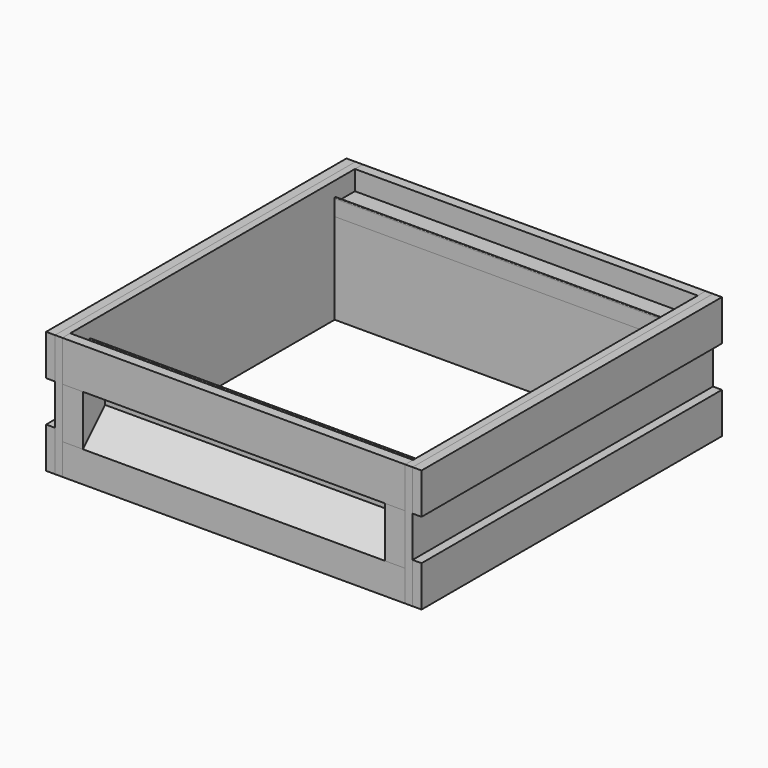
from build123d import *

# Parameters (mm, degrees)
F0_W      = 9
F0_H      = 126
F1_DEPTH  = 210
F2_W      = 34
F2_H      = 38
F3_DEPTH  = 210
F5_DEPTH  = 420
F9_DEPTH  = 9
F10_W     = 11
F10_H     = 50
F11_DEPTH = 460
F12_W     = 34
F12_H     = 62
F13_DEPTH = 25
F16_DEPTH = 370


# Not quite as in the source:
# - ends of sketch curves that miss each other by under 0.0002 mm in the source are joined


with BuildPart() as f1:
    # F0 (on Right) → F1 (new body, symmetric)
    with BuildSketch(Plane.YZ):
        with Locations((39.679, 225.9123)):
            Rectangle(F0_W, F0_H)
    extrude(amount=F1_DEPTH, both=True)


with BuildPart() as f1b:
    # F0 (on Right) → F1, piece 2 (new body, symmetric)
    with BuildSketch(Plane.YZ):
        Polygon((427.179, 288.9123), (418.179, 288.9123), (418.179, 162.9122999998), (427.1789405548, 162.9123), align=None)
    extrude(amount=F1_DEPTH, both=True)


with BuildPart() as f3:
    # F2 (on Right) → F3 (new body, symmetric)
    with BuildSketch(Plane.YZ):
        with Locations((18.179, 181.9123)):
            Rectangle(F2_W, F2_H)
    extrude(amount=F3_DEPTH, both=True)


with BuildPart() as f3b:
    # F2 (on Right) → F3, piece 2 (new body, symmetric)
    with BuildSketch(Plane.YZ):
        Polygon((13.179, 312.9123), (1.179, 312.9123), (1.179, 262.9123), (35.179, 262.9123), (35.179, 288.9123), (13.179, 288.9123), align=None)
    extrude(amount=F3_DEPTH, both=True)


with BuildPart() as f3c:
    # F2 (on Right) → F3, piece 3 (new body, symmetric)
    with BuildSketch(Plane.YZ):
        Polygon((461.179, 262.9123), (461.179, 312.9123), (449.179, 312.9123), (449.179, 288.9123), (427.179, 288.9123), (427.179, 262.9123), align=None)
    extrude(amount=F3_DEPTH, both=True)


with BuildPart() as f3d:
    # F2 (on Right) → F3, piece 4 (new body, symmetric)
    with BuildSketch(Plane.YZ):
        with Locations((444.179, 181.9123)):
            Rectangle(F2_W, F2_H)
    extrude(amount=F3_DEPTH, both=True)


with BuildPart() as f5:
    # F4 (on face) → F5 (new body, through all)
    with BuildSketch(Plane.YZ.offset(210)):
        with BuildLine():
            ThreePointArc((43.1172127334, 294.2653739331), (43.7826266683, 294.4466811128), (44.179, 293.8822910173))
            Line((44.179, 293.8822910173), (44.179, 274.5153307915))
            Line((44.179, 274.5153307915), (44.729, 274.5153307915))
            Line((44.729, 274.5153307915), (44.729, 293.8822910173))
            ThreePointArc((44.729, 293.8822910173), (44.4858001945, 294.5895486841), (43.8590636395, 294.9976673474))
            Line((43.8590636395, 294.9976673474), (43.2989363605, 294.9976673474))
            ThreePointArc((43.2989363605, 294.9976673474), (42.9660457898, 294.8553208915), (42.6939077391, 294.6165332727))
            Line((42.6939077391, 294.6165332727), (38.2546330976, 289.2652100541))
            Line((38.2546330976, 289.2652100541), (38.679, 288.9153307915))
            Line((38.679, 288.9153307915), (43.1172127334, 294.2653739331))
        make_face()
    extrude(amount=-F5_DEPTH)


with BuildPart() as f7_1:
    # F7: instance of F5
    add(f5.part.mirror(Plane(origin=(0, 231.179, 225.9122999999), x_dir=(-1, 0, 0), z_dir=(0, 1, 0))))


with BuildPart() as f9:
    # F8 (on face) → F9 (new body)
    with BuildSketch(Plane.YZ.offset(210)):
        Polygon((1.179, 312.9123), (1.179, 162.9123), (461.179, 162.9123), (461.179, 312.9123), (13.179, 312.9123), align=None)
    extrude(amount=F9_DEPTH)


with BuildPart() as f11:
    # F10 (on face) → F11 (new body, through all)
    with BuildSketch(Plane.XZ.offset(-1.179)):
        with Locations((224.5, 287.9123)):
            Rectangle(F10_W, F10_H)
    extrude(amount=-F11_DEPTH)


with BuildPart() as f11b:
    # F10 (on face) → F11, piece 2 (new body, through all)
    with BuildSketch(Plane.XZ.offset(-1.179)):
        with Locations((224.5, 187.9123)):
            Rectangle(F10_W, F10_H)
    extrude(amount=-F11_DEPTH)


with BuildPart() as f13:
    # F12 (on face) → F13 (new body)
    with BuildSketch(Plane(origin=(210, 0, 0), x_dir=(0, -1, 0), z_dir=(-1, 0, 0))):
        with Locations((-18.179, 231.9123)):
            Rectangle(F12_W, F12_H)
    extrude(amount=F13_DEPTH)


with BuildPart() as f13b:
    # F12 (on face) → F13, piece 2 (new body)
    with BuildSketch(Plane(origin=(210, 0, 0), x_dir=(0, -1, 0), z_dir=(-1, 0, 0))):
        with Locations((-444.179, 231.9123)):
            Rectangle(F12_W, F12_H)
    extrude(amount=F13_DEPTH)


with BuildPart() as f14_1:
    # F14: instance of F9
    add(f9.part.mirror(Plane.YZ))


with BuildPart() as f14_2:
    # F14: instance of F11b
    add(f11b.part.mirror(Plane.YZ))


with BuildPart() as f14_3:
    # F14: instance of F11
    add(f11.part.mirror(Plane.YZ))


with BuildPart() as f14_4:
    # F14: instance of F13
    add(f13.part.mirror(Plane.YZ))


with BuildPart() as f14_5:
    # F14: instance of F13b
    add(f13b.part.mirror(Plane.YZ))


with BuildPart() as f16:
    # F15 (on face) → F16 (new body, through all)
    with BuildSketch(Plane(origin=(185, 0, 0), x_dir=(0, -1, 0), z_dir=(-1, 0, 0))):
        Polygon((-35.179, 234.9123), (-35.179, 200.9123), (-1.179, 200.9123), align=None)
    extrude(amount=F16_DEPTH)


with BuildPart() as f16b:
    # F15 (on face) → F16, piece 2 (new body, through all)
    with BuildSketch(Plane(origin=(185, 0, 0), x_dir=(0, -1, 0), z_dir=(-1, 0, 0))):
        Polygon((-461.179, 200.9123), (-427.179, 200.9123), (-427.179, 234.9123), align=None)
    extrude(amount=F16_DEPTH)


solid = Compound([f1.part, f1b.part, f3.part, f3b.part, f3c.part, f3d.part, f5.part, f7_1.part, f9.part, f11.part, f11b.part, f13.part, f13b.part, f14_1.part, f14_2.part, f14_3.part, f14_4.part, f14_5.part, f16.part, f16b.part])
